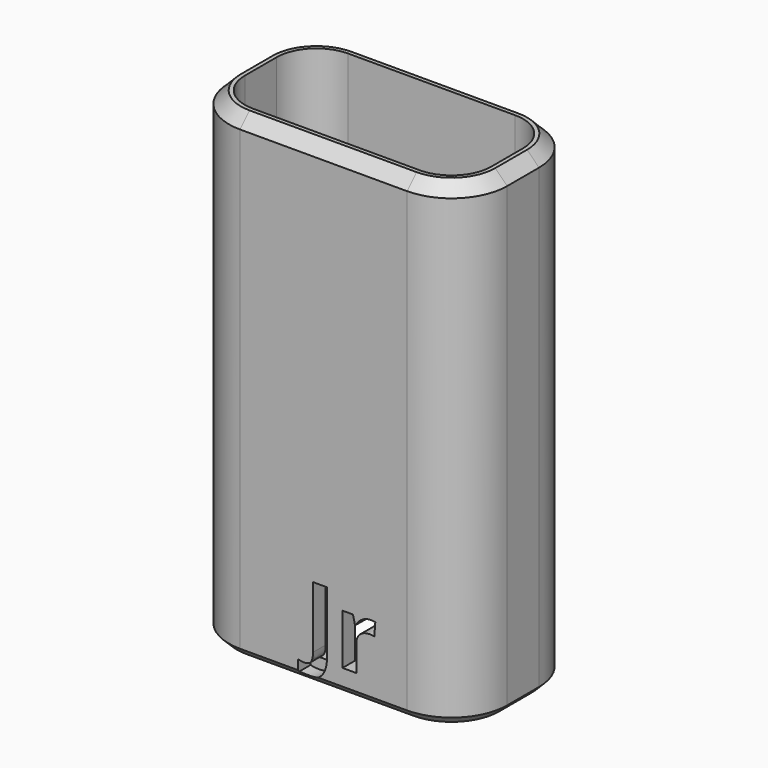
from build123d import *

# Parameters (mm, degrees)
F0_W         = 27
F0_H         = 11
F1_DEPTH     = 2
F2_DEPTH     = 60
F3_W         = 7
F3_H         = 4
F4_DEPTH     = 25
F5_TEXT_SIZE = 11.6242864556
F6_DEPTH     = 25
F7_T1_DEPTH  = 21
F7_T3_DEPTH  = 5
F7_T6_ANGLE  = 90
F7_T8_ANGLE  = 90
F7_T10_ANGLE = 90
F7_T12_ANGLE = 90
F8_SIZE      = 1.5


# Not quite as in the source:
# - a fillet or chamfer that OpenCascade refuses, or shapes differently, is made with other operations: its cross-section is extruded or revolved along the edge and cut away or added
# - Text() gives the source's letters only with a copy of the font that has no kerning and outlines rounded to 1/6400 em; it was checked with that copy


with BuildPart() as f1:
    # F0 (on Top) → F1 (new body)
    with BuildSketch(Plane.XY):
        with BuildLine():
            Line((26, 17), (5, 17))
            ThreePointArc((5, 17), (0.0502525317, 14.9497474683), (-2, 10))
            Line((-2, 10), (-2, 5))
            ThreePointArc((-2, 5), (0.0502525317, 0.0502525317), (5, -2))
            Line((5, -2), (26, -2))
            ThreePointArc((26, -2), (30.9497474683, 0.0502525317), (33, 5))
            Line((33, 5), (33, 10))
            ThreePointArc((33, 10), (30.9497474683, 14.9497474683), (26, 17))
        make_face()
        with BuildLine():
            Line((26, 0), (5, 0))
            ThreePointArc((5, 0), (1.4644660941, 1.4644660941), (0, 5))
            Line((0, 5), (0, 10))
            ThreePointArc((0, 10), (1.4644660941, 13.5355339059), (5, 15))
            Line((5, 15), (26, 15))
            ThreePointArc((26, 15), (29.5355339059, 13.5355339059), (31, 10))
            Line((31, 10), (31, 5))
            ThreePointArc((31, 5), (29.5355339059, 1.4644660941), (26, 0))
        make_face(mode=Mode.SUBTRACT)
        with BuildLine():
            ThreePointArc((0, 5), (1.4644660941, 1.4644660941), (5, 0))
            Line((5, 0), (26, 0))
            ThreePointArc((26, 0), (29.5355339059, 1.4644660941), (31, 5))
            Line((31, 5), (31, 10))
            ThreePointArc((31, 10), (29.5355339059, 13.5355339059), (26, 15))
            Line((26, 15), (5, 15))
            ThreePointArc((5, 15), (1.4644660941, 13.5355339059), (0, 10))
            Line((0, 10), (0, 5))
        make_face()
        with Locations((15.5, 7.5)):
            Rectangle(F0_W, F0_H, mode=Mode.SUBTRACT)
    extrude(amount=F1_DEPTH)

    # F0 (on Top) → F2 (join)
    with BuildSketch(Plane.XY):
        with BuildLine():
            Line((26, 17), (5, 17))
            ThreePointArc((5, 17), (0.0502525317, 14.9497474683), (-2, 10))
            Line((-2, 10), (-2, 5))
            ThreePointArc((-2, 5), (0.0502525317, 0.0502525317), (5, -2))
            Line((5, -2), (26, -2))
            ThreePointArc((26, -2), (30.9497474683, 0.0502525317), (33, 5))
            Line((33, 5), (33, 10))
            ThreePointArc((33, 10), (30.9497474683, 14.9497474683), (26, 17))
        make_face()
        with BuildLine():
            Line((26, 0), (5, 0))
            ThreePointArc((5, 0), (1.4644660941, 1.4644660941), (0, 5))
            Line((0, 5), (0, 10))
            ThreePointArc((0, 10), (1.4644660941, 13.5355339059), (5, 15))
            Line((5, 15), (26, 15))
            ThreePointArc((26, 15), (29.5355339059, 13.5355339059), (31, 10))
            Line((31, 10), (31, 5))
            ThreePointArc((31, 5), (29.5355339059, 1.4644660941), (26, 0))
        make_face(mode=Mode.SUBTRACT)
    extrude(amount=F2_DEPTH)

    # F3 (on Front) → F4 (cut)
    with BuildSketch(Plane.XZ):
        with Locations((16, 27.0405690297)):
            Rectangle(F3_W, F3_H)
    extrude(amount=-F4_DEPTH, mode=Mode.SUBTRACT)

    # F5 (on Front) → F6 (cut)
    with BuildSketch(Plane.XZ):
        with Locations((13.1230571789, 3.0648915141)):
            Text('Jr', F5_TEXT_SIZE, font='Open Sans', font_style=FontStyle.BOLD, text_align=(TextAlign.LEFT, TextAlign.BOTTOM))
    extrude(amount=F6_DEPTH, mode=Mode.SUBTRACT)

    # F7: chamfer of 1 on 8 edges, made by hand

    # F7_s2 → F7_t1 (cut)
    with BuildSketch(Plane.YZ.offset(5)):
        Polygon((-1, 0), (-2, 1), (-2, 0), align=None)
        Polygon((16, 0), (17, 1), (17, 0), align=None)
    extrude(amount=F7_T1_DEPTH, mode=Mode.SUBTRACT)

    # F7_s4 → F7_t3 (cut)
    with BuildSketch(Plane.XZ.offset(-10)):
        Polygon((-1, 0), (-2, 1), (-2, 0), align=None)
        Polygon((32, 0), (33, 1), (33, 0), align=None)
    extrude(amount=F7_T3_DEPTH, mode=Mode.SUBTRACT)

    # F7_s5 → F7_t6 (revolve, cut)
    with BuildSketch(Plane.XZ.offset(-5)):
        Polygon((-1, 0), (-2, 1), (-2, 0), align=None)
    revolve(axis=Axis((5, 5, 0), (0, 0, 1)), revolution_arc=F7_T6_ANGLE, mode=Mode.SUBTRACT)

    # F7_s7 → F7_t8 (revolve, cut)
    with BuildSketch(Plane.YZ.offset(5)):
        Polygon((16, 0), (17, 1), (17, 0), align=None)
    revolve(axis=Axis((5, 10, 0), (0, 0, 1)), revolution_arc=F7_T8_ANGLE, mode=Mode.SUBTRACT)

    # F7_s9 → F7_t10 (revolve, cut)
    with BuildSketch(Plane.XZ.offset(-10)):
        Polygon((32, 0), (33, 1), (33, 0), align=None)
    revolve(axis=Axis((26, 10, 0), (0, 0, 1)), revolution_arc=F7_T10_ANGLE, mode=Mode.SUBTRACT)

    # F7_s11 → F7_t12 (revolve, cut)
    with BuildSketch(Plane.YZ.offset(26)):
        Polygon((-1, 0), (-2, 1), (-2, 0), align=None)
    revolve(axis=Axis((26, 5, 0), (0, 0, 1)), revolution_arc=F7_T12_ANGLE, mode=Mode.SUBTRACT)

    # F8
    f8_edges = [f1.edges().sort_by_distance(p)[0] for p in [
        (15.5, -2, 60),
        (30.949747, 0.050253, 60),
        (33, 7.5, 60),
        (30.949747, 14.949747, 60),
        (15.5, 17, 60),
        (0.050253, 14.949747, 60),
        (-2, 7.5, 60),
        (0.050253, 0.050253, 60),
    ]]
    chamfer(f8_edges, length=F8_SIZE)


solid = f1.part
